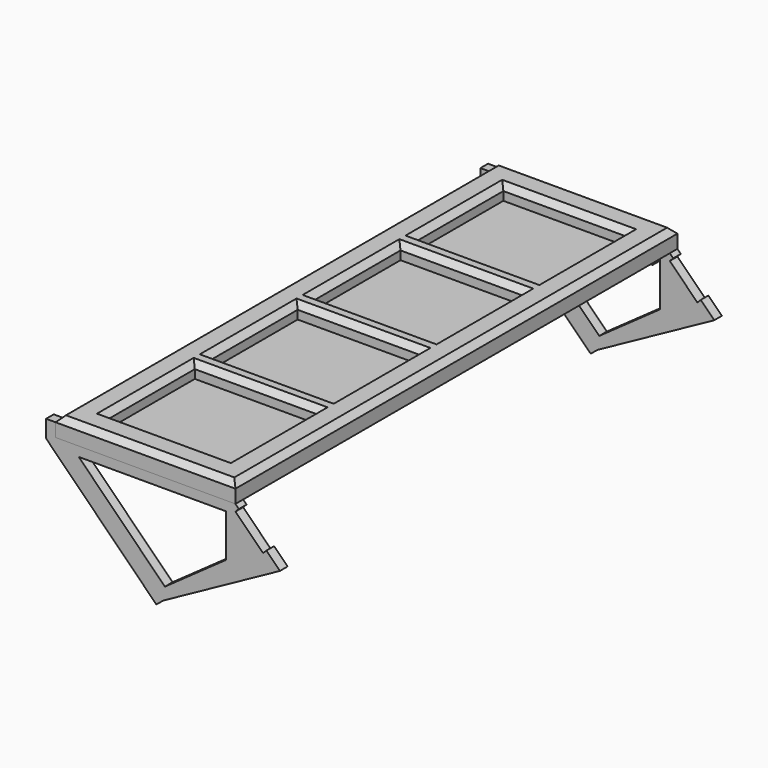
from build123d import *

# Parameters (mm, degrees)
F0_W     = 59.69
F0_H     = 183.388
F0_W_2   = 40.64
F0_H_2   = 6.35
F1_DEPTH = 6.35
F2_SIZE  = 1.905
F0_H_3   = 36.322
F3_DEPTH = 1.5875
F5_DEPTH = 3.175
F7_DEPTH = 25.4
F8_W     = 48.8498719395
F8_H     = 3.175
F9_DEPTH = 3.175


with BuildPart() as f1:
    # F0 (on Top) → F1 (new body)
    with BuildSketch(Plane.XY):
        Rectangle(F0_W, F0_H)
        Polygon((20.32, -45.847), (20.32, -82.169), (-20.32, -82.169), (-20.32, -45.847), (-20.32, -39.497), (-20.32, -3.175), (-20.32, 3.175), (-20.32, 39.497), (-20.32, 45.847), (-20.32, 82.169), (20.32, 82.169), (20.32, 45.847), (20.32, 39.497), (20.32, 3.175), (20.32, -3.175), (20.32, -39.497), align=None, mode=Mode.SUBTRACT)
        Rectangle(F0_W_2, F0_H_2)
        with Locations((0, -42.672)):
            Rectangle(F0_W_2, F0_H_2)
        with Locations((0, 42.672)):
            Rectangle(F0_W_2, F0_H_2)
    extrude(amount=F1_DEPTH)

    # F2
    f2_edges = [f1.edges().sort_by_distance(p)[0] for p in [
        (-29.845, 0, 6.35),
        (0, -91.694, 6.35),
        (29.845, 0, 6.35),
        (0, 91.694, 6.35),
        (0, -82.169, 6.35),
        (-20.32, -64.008, 6.35),
        (0, -45.847, 6.35),
        (20.32, -64.008, 6.35),
        (-20.32, -21.336, 6.35),
        (0, -3.175, 6.35),
        (20.32, -21.336, 6.35),
        (0, -39.497, 6.35),
        (-20.32, 21.336, 6.35),
        (0, 39.497, 6.35),
        (20.32, 21.336, 6.35),
        (0, 3.175, 6.35),
        (-20.32, 64.008, 6.35),
        (0, 82.169, 6.35),
        (20.32, 64.008, 6.35),
        (0, 45.847, 6.35),
    ]]
    chamfer(f2_edges, length=F2_SIZE)

    # F0 (on Top) → F3 (join)
    with BuildSketch(Plane.XY):
        with Locations((0, -64.008)):
            Rectangle(F0_W_2, F0_H_3)
        with Locations((0, -21.336)):
            Rectangle(F0_W_2, F0_H_3)
        with Locations((0, 21.336)):
            Rectangle(F0_W_2, F0_H_3)
        with Locations((0, 64.008)):
            Rectangle(F0_W_2, F0_H_3)
    extrude(amount=F3_DEPTH)


with BuildPart() as f5:
    # F4 (on face) → F5 (new body)
    with BuildSketch(Plane.XZ.offset(91.694)):
        Polygon((29.845, 0), (20.32, 0), (-20.32, 0), (-29.845, 0), (6.0760244843, -35.9210244843), (44.6175213192, -14.7725213192), (40.1273932586, -10.2823932586), (39.0048612435, -11.4049252738), (29.845, -2.2450640303), (30.9675320151, -1.1225320151), align=None)
        Polygon((6.0760244843, -35.9210244843), (-29.845, 0), (-29.845, 4.445), (-33.02, 4.445), (-33.02, -1.3151280605), (3.5546971341, -37.8898251946), align=None)
    extrude(amount=-F5_DEPTH)

    # F6 (on face) → F7 (cut)
    with BuildSketch(Plane.XZ.offset(91.694)):
        Polygon((6.424976296, -31.7798482355), (26.67, -17.4100959351), (26.67, -3.175), (-22.1798719395, -3.175), align=None)
    extrude(amount=-F7_DEPTH, mode=Mode.SUBTRACT)

    # F8 (on face) → F9 (join)
    with BuildSketch(Plane(origin=(0, -88.519, 0), x_dir=(-1, 0, 0), z_dir=(0, 1, 0))):
        with Locations((-2.2450640303, -1.5875)):
            Rectangle(F8_W, F8_H)
    extrude(amount=F9_DEPTH)


with BuildPart() as f10_1:
    # F10: instance of F5
    add(f5.part.mirror(Plane.XZ))


solid = Compound([f1.part, f5.part, f10_1.part])
